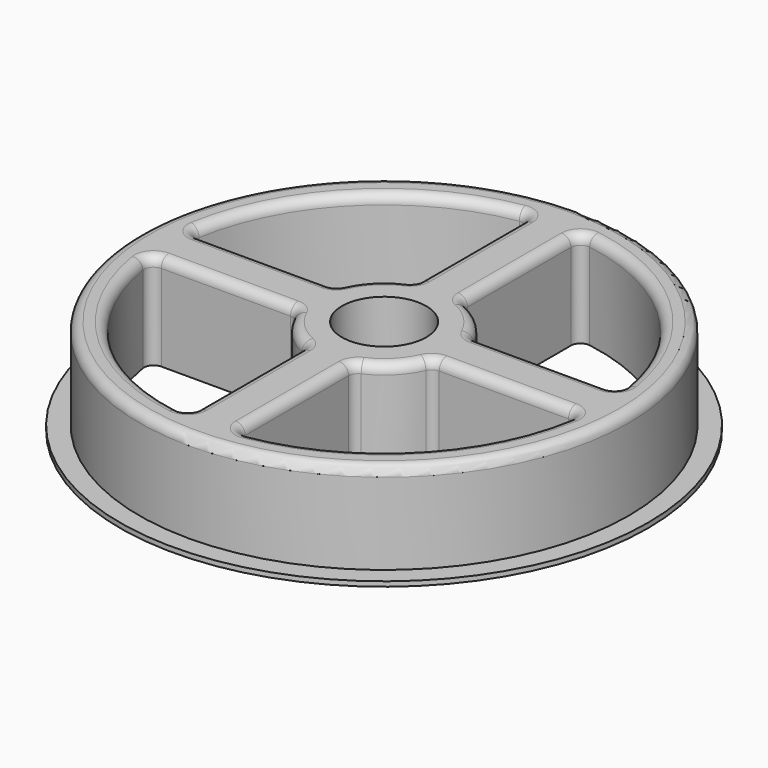
from build123d import *

# Parameters (mm, degrees)
F0_R            = 25.5
F1_DEPTH        = 10
F0_R_2          = 27.5
F2_DEPTH        = 0.5
F3_R            = 22.5
F3_R_2          = 7.5
F4_DEPTH        = 10.001
F6_DEPTH        = 10
F6_COPIES_COUNT = 4
F7_R            = 1
F8_R            = 4.4
F9_DEPTH        = 10.001


# Not quite as in the source:
# - a pattern or mirror of a feature is missing from the dataset's text; its kind, count and spacing are read off the source's solid


with BuildPart() as f1:
    # F0 (on Top) → F1 (new body)
    with BuildSketch(Plane.XY):
        Circle(F0_R)
    extrude(amount=F1_DEPTH)

    # F0 (on Top) → F2 (join)
    with BuildSketch(Plane.XY):
        Circle(F0_R_2)
        Circle(F0_R, mode=Mode.SUBTRACT)
    extrude(amount=F2_DEPTH)

    # F3 (on face) → F4 (cut, through all)
    with BuildSketch(Plane.XY.offset(10)):
        Circle(F3_R)
        Circle(F3_R_2, mode=Mode.SUBTRACT)
    extrude(amount=-F4_DEPTH, mode=Mode.SUBTRACT)

    # F5 (on face) → F6 (join, through all)
    with BuildSketch(Plane.XY.offset(10)):
        with BuildLine():
            Line((7.0710678119, -2.5), (22.5, -2.5))
            Line((22.5, -2.5), (22.5, 2.5))
            Line((22.5, 2.5), (7.0710678119, 2.5))
            ThreePointArc((7.0710678119, 2.5), (7.3919891974, 1.2682648404), (7.5, 0))
            ThreePointArc((7.5, 0), (7.3919891974, -1.2682648404), (7.0710678119, -2.5))
        make_face()
    f6 = extrude(amount=-F6_DEPTH)

    # F6_copies: F6 ×4 about axis
    f6_copies_axis = Axis((0, 0, 0), (0, 0, 1))
    for i in range(1, F6_COPIES_COUNT):
        add(f6.rotate(f6_copies_axis, i * 360 / F6_COPIES_COUNT))

    # F7
    f7_edges = [f1.edges().sort_by_distance(p)[0] for p in [
        (-15.909903, -15.909903, 10),
        (15.909903, -15.909903, 10),
        (-15.909903, 15.909903, 10),
        (15.909903, 15.909903, 10),
        (14.715874, 2.5, 10),
        (-5.303301, -5.303301, 10),
        (5.303301, -5.303301, 10),
        (-5.303301, 5.303301, 10),
        (5.303301, 5.303301, 10),
        (14.715874, -2.5, 10),
        (-25.5, 0, 10),
        (-14.715874, -2.5, 10),
        (-2.5, -14.715874, 10),
        (2.5, -14.715874, 10),
        (-2.5, 14.715874, 10),
        (-14.715874, 2.5, 10),
        (2.5, 14.715874, 10),
        (-2.5, -22.36068, 5),
        (-22.36068, -2.5, 5),
        (22.36068, -2.5, 5),
        (2.5, -22.36068, 5),
        (7.071068, -2.5, 5),
        (2.5, -7.071068, 5),
        (-2.5, -7.071068, 5),
        (-7.071068, -2.5, 5),
        (-22.36068, 2.5, 5),
        (-2.5, 22.36068, 5),
        (-2.5, 7.071068, 5),
        (-7.071068, 2.5, 5),
        (2.5, 22.36068, 5),
        (22.36068, 2.5, 5),
        (7.071068, 2.5, 5),
        (2.5, 7.071068, 5),
    ]]
    fillet(f7_edges, radius=F7_R)

    # F8 (on face) → F9 (cut, through all)
    with BuildSketch(Plane.XY.offset(10)):
        Circle(F8_R)
    extrude(amount=-F9_DEPTH, mode=Mode.SUBTRACT)


solid = f1.part
